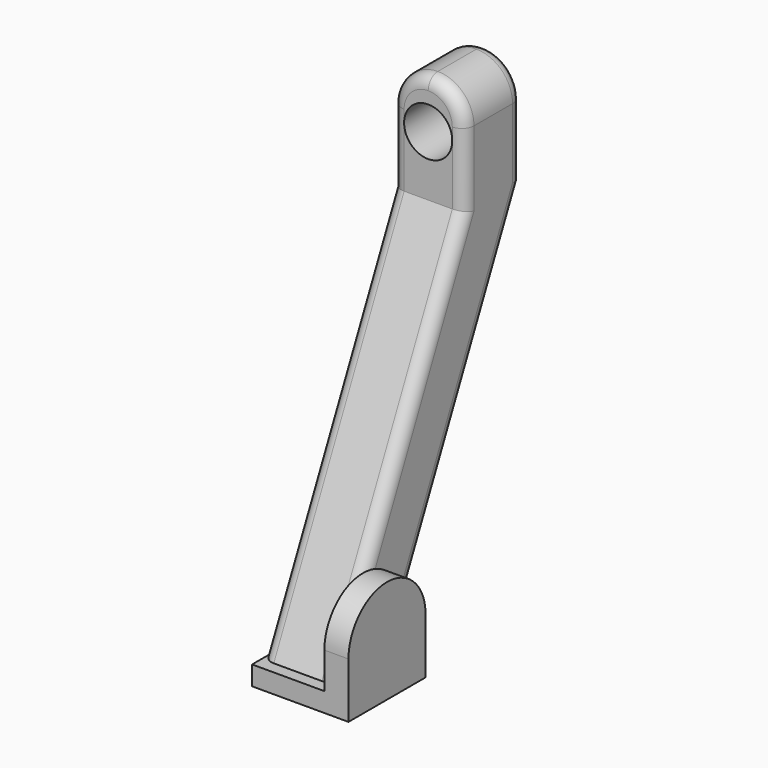
from build123d import *

# Parameters (mm, degrees)
F0_W      = 4
F0_H      = 4
F1_DEPTH  = 0.8
F4_DEPTH  = 1.5
F5_R      = 1
F6_DEPTH  = 10.2624610432
F7_R      = 1.49999
F8_R      = 0.49999
F10_DEPTH = 1


# Not quite as in the source:
# - a fillet or chamfer is up to 0.001 mm smaller than in the source, because OpenCascade refuses the exact size


with BuildPart() as f1:
    # F0 (on Top) → F1 (new body)
    with BuildSketch(Plane.XY):
        with Locations((3, 2)):
            Rectangle(F0_W, F0_H)
    extrude(amount=F1_DEPTH)

    # F3 (on offset) → F4 (join, symmetric)
    with BuildSketch(Plane.YZ.offset(2.5)):
        Polygon((0.5, 0.8), (3.5, 0.8), (10.2614610432, 15.3), (10.2614610432, 19.8), (7.2614610432, 19.8), (7.2614610432, 15.3), align=None)
    extrude(amount=F4_DEPTH, both=True)

    # F5 (on face) → F6 (cut, through all)
    with BuildSketch(Plane(origin=(0, 10.2614610432, 0), x_dir=(-1, 0, 0), z_dir=(0, 1, 0))):
        with Locations((-2.5, 17.8)):
            Circle(F5_R)
    extrude(amount=-F6_DEPTH, mode=Mode.SUBTRACT)

    # F7 (radius 1.5 in the source; OpenCascade refuses exactly that, so slightly less here)
    f7_edges = [f1.edges().sort_by_distance(p)[0] for p in [
        (1, 8.761461, 19.8),
        (4, 8.761461, 19.8),
    ]]
    fillet(f7_edges, radius=F7_R)

    # F8 (radius 0.5 in the source; OpenCascade refuses exactly that, so slightly less here)
    f8_edges = [f1.edges().sort_by_distance(p)[0] for p in [
        (1, 6.880731, 8.05),
        (1, 10.261461, 16.800005),
        (3.560663, 10.261461, 19.360663),
        (4, 6.880731, 8.05),
        (1, 3.880731, 8.05),
        (1, 7.261461, 16.800005),
        (4, 3.880731, 8.05),
    ]]
    fillet(f8_edges, radius=F8_R)

    # F9 (on face) → F10 (join)
    with BuildSketch(Plane.YZ.offset(5)):
        with BuildLine():
            Line((0, 2.3), (0, 0.8))
            Line((0, 0.8), (4, 0.8))
            Line((4, 0.8), (4, 2.3))
            ThreePointArc((4, 2.3), (2, 4.3), (0, 2.3))
        make_face()
    extrude(amount=-F10_DEPTH)


solid = f1.part
